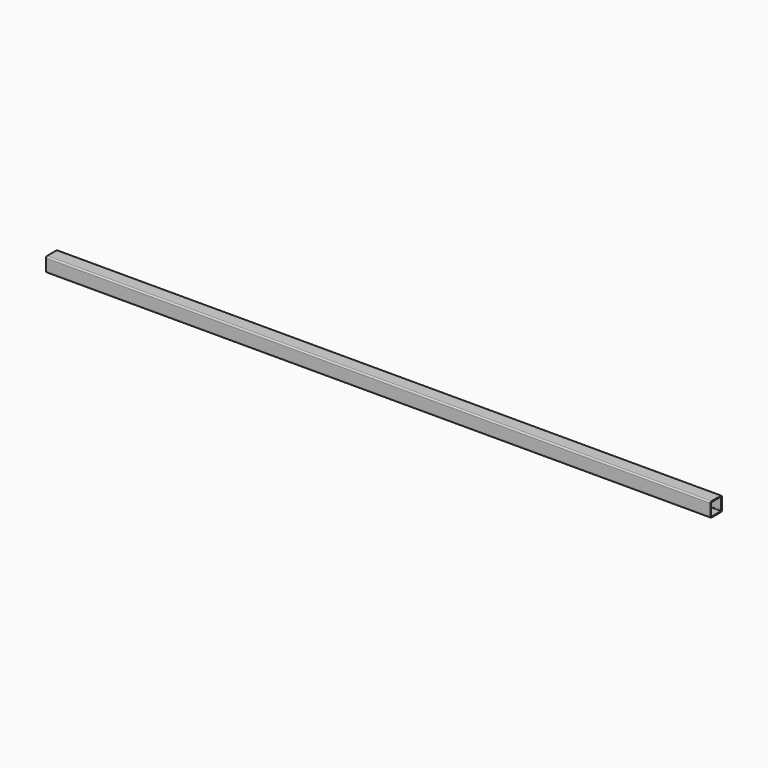
from build123d import *

# Parameters (mm, degrees)
F0_W     = 50.8
F0_H     = 50.8
F1_DEPTH = 1168.4
F2_T     = -3.175
F3_R     = 4.7625
F4_R     = 2.38125


with BuildPart() as f1:
    # F0 (on Right) → F1 (new body, symmetric)
    with BuildSketch(Plane.YZ):
        Rectangle(F0_W, F0_H)
    extrude(amount=F1_DEPTH, both=True)

    # F2
    f2_openings = [f1.faces().sort_by_distance(p)[0] for p in [
        (1168.4, 0, 0),
        (-1168.4, 0, 0),
    ]]
    offset(amount=F2_T, openings=f2_openings)

    # F3
    f3_edges = [f1.edges().sort_by_distance(p)[0] for p in [
        (0, 25.4, 25.4),
        (0, -25.4, 25.4),
        (0, 25.4, -25.4),
        (0, -25.4, -25.4),
    ]]
    fillet(f3_edges, radius=F3_R)

    # F4
    f4_edges = [f1.edges().sort_by_distance(p)[0] for p in [
        (0, -22.225, 22.225),
        (0, -22.225, -22.225),
        (0, 22.225, -22.225),
        (0, 22.225, 22.225),
    ]]
    fillet(f4_edges, radius=F4_R)


solid = f1.part
